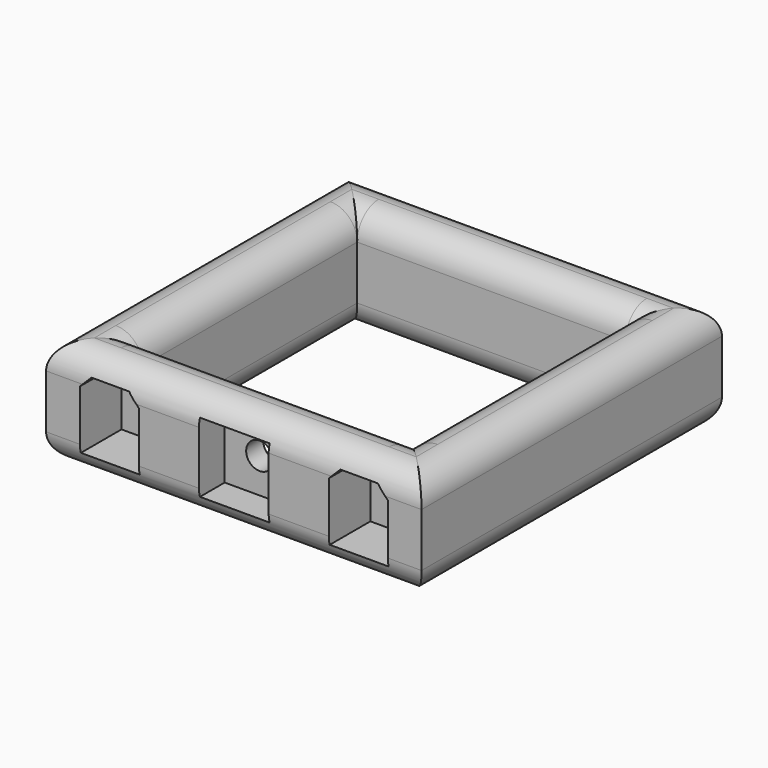
from build123d import *

# Parameters (mm, degrees)
F0_W         = 70
F0_H         = 70
F0_W_2       = 50
F0_H_2       = 50
F1_DEPTH     = 20
F2_W         = 13
F2_H         = 13
F3_DEPTH     = 6
F4_T1_DEPTH  = 95
F4_T3_DEPTH  = 95
F4_T5_DEPTH  = 50
F4_T7_DEPTH  = 50
F4_T13_DEPTH = 62.5
F4_T17_DEPTH = 62.5
F4_T24_DEPTH = 62.5
F4_T28_DEPTH = 62.5
F4_T35_DEPTH = 62.5
F4_T39_DEPTH = 62.5
F4_T46_DEPTH = 62.5
F4_T50_DEPTH = 62.5
F4_T57_DEPTH = 62.5
F4_T61_DEPTH = 62.5
F4_T68_DEPTH = 62.5
F4_T72_DEPTH = 62.5
F4_T79_DEPTH = 62.5
F4_T83_DEPTH = 62.5
F4_T90_DEPTH = 62.5
F4_T94_DEPTH = 62.5
F5_R         = 2.5
F6_DEPTH     = 25
F7_W         = 11
F7_H         = 13
F8_DEPTH     = 9.7
F9_SIZE      = 2
F10_SIZE     = 2


# Not quite as in the source:
# - a fillet or chamfer that OpenCascade refuses, or shapes differently, is made with other operations: its cross-section is extruded or revolved along the edge and cut away or added


with BuildPart() as f1:
    # F0 (on Top) → F1 (new body)
    with BuildSketch(Plane.XY):
        with Locations((7.0071799593, -0.6538340822)):
            Rectangle(F0_W, F0_H)
        with Locations((7.0071799593, -0.6538340822)):
            Rectangle(F0_W_2, F0_H_2, mode=Mode.SUBTRACT)
    extrude(amount=F1_DEPTH)

    # F2 (on face) → F3 (cut)
    with BuildSketch(Plane.XZ.offset(35.6538340822)):
        with Locations((7.0071799593, 10)):
            Rectangle(F2_W, F2_H)
    extrude(amount=-F3_DEPTH, mode=Mode.SUBTRACT)

    # F4: fillet of radius 5 on 16 edges, made by hand

    # F4_s2 → F4_t1 (cut)
    with BuildSketch(Plane.XZ.offset(-46.8461659178)):
        with BuildLine():
            ThreePointArc((42.0071799593, 5), (40.5427138653, 1.4644660941), (37.0071799593, 0))
            Line((37.0071799593, 0), (42.0071799593, 0))
            Line((42.0071799593, 0), (42.0071799593, 5))
        make_face()
        with BuildLine():
            ThreePointArc((42.0071799593, 15), (40.5427138653, 18.5355339059), (37.0071799593, 20))
            Line((37.0071799593, 20), (42.0071799593, 20))
            Line((42.0071799593, 20), (42.0071799593, 15))
        make_face()
        with BuildLine():
            ThreePointArc((-22.9928200407, 0), (-26.5283539466, 1.4644660941), (-27.9928200407, 5))
            Line((-27.9928200407, 5), (-27.9928200407, 0))
            Line((-27.9928200407, 0), (-22.9928200407, 0))
        make_face()
        with BuildLine():
            ThreePointArc((-22.9928200407, 20), (-26.5283539466, 18.5355339059), (-27.9928200407, 15))
            Line((-27.9928200407, 15), (-27.9928200407, 20))
            Line((-27.9928200407, 20), (-22.9928200407, 20))
        make_face()
    extrude(amount=F4_T1_DEPTH, mode=Mode.SUBTRACT)

    # F4_s4 → F4_t3 (cut)
    with BuildSketch(Plane.YZ.offset(-40.4928200407)):
        with BuildLine():
            ThreePointArc((-35.6538340822, 5), (-34.1893679881, 1.4644660941), (-30.6538340822, 0))
            Line((-30.6538340822, 0), (-35.6538340822, 0))
            Line((-35.6538340822, 0), (-35.6538340822, 5))
        make_face()
        with BuildLine():
            ThreePointArc((-35.6538340822, 15), (-34.1893679881, 18.5355339059), (-30.6538340822, 20))
            Line((-30.6538340822, 20), (-35.6538340822, 20))
            Line((-35.6538340822, 20), (-35.6538340822, 15))
        make_face()
        with BuildLine():
            ThreePointArc((34.3461659178, 5), (32.8816998237, 1.4644660941), (29.3461659178, 0))
            Line((29.3461659178, 0), (34.3461659178, 0))
            Line((34.3461659178, 0), (34.3461659178, 5))
        make_face()
        with BuildLine():
            ThreePointArc((34.3461659178, 15), (32.8816998237, 18.5355339059), (29.3461659178, 20))
            Line((29.3461659178, 20), (34.3461659178, 20))
            Line((34.3461659178, 20), (34.3461659178, 15))
        make_face()
    extrude(amount=F4_T3_DEPTH, mode=Mode.SUBTRACT)

    # F4_s6 → F4_t5 (cut)
    with BuildSketch(Plane.XZ.offset(-24.3461659178)):
        with BuildLine():
            ThreePointArc((-22.9928200407, 0), (-19.4572861347, 1.4644660941), (-17.9928200407, 5))
            Line((-17.9928200407, 5), (-17.9928200407, 0))
            Line((-17.9928200407, 0), (-22.9928200407, 0))
        make_face()
        with BuildLine():
            ThreePointArc((37.0071799593, 0), (33.4716460534, 1.4644660941), (32.0071799593, 5))
            Line((32.0071799593, 5), (32.0071799593, 0))
            Line((32.0071799593, 0), (37.0071799593, 0))
        make_face()
        with BuildLine():
            ThreePointArc((-22.9928200407, 20), (-19.4572861347, 18.5355339059), (-17.9928200407, 15))
            Line((-17.9928200407, 15), (-17.9928200407, 20))
            Line((-17.9928200407, 20), (-22.9928200407, 20))
        make_face()
        with BuildLine():
            ThreePointArc((37.0071799593, 20), (33.4716460534, 18.5355339059), (32.0071799593, 15))
            Line((32.0071799593, 15), (32.0071799593, 20))
            Line((32.0071799593, 20), (37.0071799593, 20))
        make_face()
    extrude(amount=F4_T5_DEPTH, mode=Mode.SUBTRACT)

    # F4_s8 → F4_t7 (cut)
    with BuildSketch(Plane.YZ.offset(-17.9928200407)):
        with BuildLine():
            ThreePointArc((29.3461659178, 0), (25.8106320119, 1.4644660941), (24.3461659178, 5))
            Line((24.3461659178, 5), (24.3461659178, 0))
            Line((24.3461659178, 0), (29.3461659178, 0))
        make_face()
        with BuildLine():
            ThreePointArc((-30.6538340822, 0), (-27.1183001763, 1.4644660941), (-25.6538340822, 5))
            Line((-25.6538340822, 5), (-25.6538340822, 0))
            Line((-25.6538340822, 0), (-30.6538340822, 0))
        make_face()
        with BuildLine():
            ThreePointArc((29.3461659178, 20), (25.8106320119, 18.5355339059), (24.3461659178, 15))
            Line((24.3461659178, 15), (24.3461659178, 20))
            Line((24.3461659178, 20), (29.3461659178, 20))
        make_face()
        with BuildLine():
            ThreePointArc((-30.6538340822, 20), (-27.1183001763, 18.5355339059), (-25.6538340822, 15))
            Line((-25.6538340822, 15), (-25.6538340822, 20))
            Line((-25.6538340822, 20), (-30.6538340822, 20))
        make_face()
    extrude(amount=F4_T7_DEPTH, mode=Mode.SUBTRACT)


with BuildPart() as f4_tool11:
    # F4_s12 → F4_t13 (new body)
    with BuildSketch(Plane.XZ.offset(38.1538340822)):
        with BuildLine():
            ThreePointArc((-22.9928200407, 0), (-19.4572861347, 1.4644660941), (-17.9928200407, 5))
            Line((-17.9928200407, 5), (-17.9928200407, 0))
            Line((-17.9928200407, 0), (-22.9928200407, 0))
        make_face()
    extrude(amount=-F4_T13_DEPTH)

    split(bisect_by=Plane.XZ.offset(25.6538340822), keep=Keep.TOP)


with BuildPart() as f4_tool15:
    # F4_s16 → F4_t17 (new body)
    with BuildSketch(Plane.YZ.offset(32.0071799593)):
        with BuildLine():
            ThreePointArc((-30.6538340822, 0), (-27.1183001763, 1.4644660941), (-25.6538340822, 5))
            Line((-25.6538340822, 5), (-25.6538340822, 0))
            Line((-25.6538340822, 0), (-30.6538340822, 0))
        make_face()
    extrude(amount=-F4_T17_DEPTH)

    split(bisect_by=Plane.YZ.offset(-17.9928200407), keep=Keep.BOTTOM)


with BuildPart() as f4_tool11_1:
    add(f4_tool11.part)

    # F4_t19: intersect F4_tool15
    add(f4_tool15.part, mode=Mode.INTERSECT)


with BuildPart() as f1_1:
    add(f1.part)

    # F4_t9: cut F4_tool11
    add(f4_tool11_1.part, mode=Mode.SUBTRACT)


with BuildPart() as f4_tool22:
    # F4_s23 → F4_t24 (new body)
    with BuildSketch(Plane.XZ.offset(25.6538340822)):
        with BuildLine():
            ThreePointArc((-22.9928200407, 0), (-19.4572861347, 1.4644660941), (-17.9928200407, 5))
            Line((-17.9928200407, 5), (-17.9928200407, 0))
            Line((-17.9928200407, 0), (-22.9928200407, 0))
        make_face()
    extrude(amount=-F4_T24_DEPTH)

    split(bisect_by=Plane.XZ.offset(-24.3461659178), keep=Keep.BOTTOM)


with BuildPart() as f4_tool26:
    # F4_s27 → F4_t28 (new body)
    with BuildSketch(Plane.YZ.offset(-30.4928200407)):
        with BuildLine():
            ThreePointArc((29.3461659178, 0), (25.8106320119, 1.4644660941), (24.3461659178, 5))
            Line((24.3461659178, 5), (24.3461659178, 0))
            Line((24.3461659178, 0), (29.3461659178, 0))
        make_face()
    extrude(amount=F4_T28_DEPTH)

    split(bisect_by=Plane.YZ.offset(-17.9928200407), keep=Keep.BOTTOM)


with BuildPart() as f4_tool22_1:
    add(f4_tool22.part)

    # F4_t30: intersect F4_tool26
    add(f4_tool26.part, mode=Mode.INTERSECT)


with BuildPart() as f1_2:
    add(f1_1.part)

    # F4_t20: cut F4_tool22
    add(f4_tool22_1.part, mode=Mode.SUBTRACT)


with BuildPart() as f4_tool33:
    # F4_s34 → F4_t35 (new body)
    with BuildSketch(Plane.YZ.offset(-17.9928200407)):
        with BuildLine():
            ThreePointArc((29.3461659178, 0), (25.8106320119, 1.4644660941), (24.3461659178, 5))
            Line((24.3461659178, 5), (24.3461659178, 0))
            Line((24.3461659178, 0), (29.3461659178, 0))
        make_face()
    extrude(amount=F4_T35_DEPTH)

    split(bisect_by=Plane.YZ.offset(32.0071799593), keep=Keep.TOP)


with BuildPart() as f4_tool37:
    # F4_s38 → F4_t39 (new body)
    with BuildSketch(Plane.XZ.offset(-36.8461659178)):
        with BuildLine():
            ThreePointArc((37.0071799593, 0), (33.4716460534, 1.4644660941), (32.0071799593, 5))
            Line((32.0071799593, 5), (32.0071799593, 0))
            Line((32.0071799593, 0), (37.0071799593, 0))
        make_face()
    extrude(amount=F4_T39_DEPTH)

    split(bisect_by=Plane.XZ.offset(-24.3461659178), keep=Keep.BOTTOM)


with BuildPart() as f4_tool33_1:
    add(f4_tool33.part)

    # F4_t41: intersect F4_tool37
    add(f4_tool37.part, mode=Mode.INTERSECT)


with BuildPart() as f1_3:
    add(f1_2.part)

    # F4_t31: cut F4_tool33
    add(f4_tool33_1.part, mode=Mode.SUBTRACT)


with BuildPart() as f4_tool44:
    # F4_s45 → F4_t46 (new body)
    with BuildSketch(Plane.XZ.offset(-24.3461659178)):
        with BuildLine():
            ThreePointArc((37.0071799593, 0), (33.4716460534, 1.4644660941), (32.0071799593, 5))
            Line((32.0071799593, 5), (32.0071799593, 0))
            Line((32.0071799593, 0), (37.0071799593, 0))
        make_face()
    extrude(amount=F4_T46_DEPTH)

    split(bisect_by=Plane.XZ.offset(25.6538340822), keep=Keep.TOP)


with BuildPart() as f4_tool48:
    # F4_s49 → F4_t50 (new body)
    with BuildSketch(Plane.YZ.offset(44.5071799593)):
        with BuildLine():
            ThreePointArc((-30.6538340822, 0), (-27.1183001763, 1.4644660941), (-25.6538340822, 5))
            Line((-25.6538340822, 5), (-25.6538340822, 0))
            Line((-25.6538340822, 0), (-30.6538340822, 0))
        make_face()
    extrude(amount=-F4_T50_DEPTH)

    split(bisect_by=Plane.YZ.offset(32.0071799593), keep=Keep.TOP)


with BuildPart() as f4_tool44_1:
    add(f4_tool44.part)

    # F4_t52: intersect F4_tool48
    add(f4_tool48.part, mode=Mode.INTERSECT)


with BuildPart() as f1_4:
    add(f1_3.part)

    # F4_t42: cut F4_tool44
    add(f4_tool44_1.part, mode=Mode.SUBTRACT)


with BuildPart() as f4_tool55:
    # F4_s56 → F4_t57 (new body)
    with BuildSketch(Plane.XZ.offset(38.1538340822)):
        with BuildLine():
            ThreePointArc((-22.9928200407, 20), (-19.4572861347, 18.5355339059), (-17.9928200407, 15))
            Line((-17.9928200407, 15), (-17.9928200407, 20))
            Line((-17.9928200407, 20), (-22.9928200407, 20))
        make_face()
    extrude(amount=-F4_T57_DEPTH)

    split(bisect_by=Plane.XZ.offset(25.6538340822), keep=Keep.TOP)


with BuildPart() as f4_tool59:
    # F4_s60 → F4_t61 (new body)
    with BuildSketch(Plane.YZ.offset(32.0071799593)):
        with BuildLine():
            ThreePointArc((-30.6538340822, 20), (-27.1183001763, 18.5355339059), (-25.6538340822, 15))
            Line((-25.6538340822, 15), (-25.6538340822, 20))
            Line((-25.6538340822, 20), (-30.6538340822, 20))
        make_face()
    extrude(amount=-F4_T61_DEPTH)

    split(bisect_by=Plane.YZ.offset(-17.9928200407), keep=Keep.BOTTOM)


with BuildPart() as f4_tool55_1:
    add(f4_tool55.part)

    # F4_t63: intersect F4_tool59
    add(f4_tool59.part, mode=Mode.INTERSECT)


with BuildPart() as f1_5:
    add(f1_4.part)

    # F4_t53: cut F4_tool55
    add(f4_tool55_1.part, mode=Mode.SUBTRACT)


with BuildPart() as f4_tool66:
    # F4_s67 → F4_t68 (new body)
    with BuildSketch(Plane.XZ.offset(25.6538340822)):
        with BuildLine():
            ThreePointArc((-22.9928200407, 20), (-19.4572861347, 18.5355339059), (-17.9928200407, 15))
            Line((-17.9928200407, 15), (-17.9928200407, 20))
            Line((-17.9928200407, 20), (-22.9928200407, 20))
        make_face()
    extrude(amount=-F4_T68_DEPTH)

    split(bisect_by=Plane.XZ.offset(-24.3461659178), keep=Keep.BOTTOM)


with BuildPart() as f4_tool70:
    # F4_s71 → F4_t72 (new body)
    with BuildSketch(Plane.YZ.offset(-30.4928200407)):
        with BuildLine():
            ThreePointArc((29.3461659178, 20), (25.8106320119, 18.5355339059), (24.3461659178, 15))
            Line((24.3461659178, 15), (24.3461659178, 20))
            Line((24.3461659178, 20), (29.3461659178, 20))
        make_face()
    extrude(amount=F4_T72_DEPTH)

    split(bisect_by=Plane.YZ.offset(-17.9928200407), keep=Keep.BOTTOM)


with BuildPart() as f4_tool66_1:
    add(f4_tool66.part)

    # F4_t74: intersect F4_tool70
    add(f4_tool70.part, mode=Mode.INTERSECT)


with BuildPart() as f1_6:
    add(f1_5.part)

    # F4_t64: cut F4_tool66
    add(f4_tool66_1.part, mode=Mode.SUBTRACT)


with BuildPart() as f4_tool77:
    # F4_s78 → F4_t79 (new body)
    with BuildSketch(Plane.YZ.offset(-17.9928200407)):
        with BuildLine():
            ThreePointArc((29.3461659178, 20), (25.8106320119, 18.5355339059), (24.3461659178, 15))
            Line((24.3461659178, 15), (24.3461659178, 20))
            Line((24.3461659178, 20), (29.3461659178, 20))
        make_face()
    extrude(amount=F4_T79_DEPTH)

    split(bisect_by=Plane.YZ.offset(32.0071799593), keep=Keep.TOP)


with BuildPart() as f4_tool81:
    # F4_s82 → F4_t83 (new body)
    with BuildSketch(Plane.XZ.offset(-36.8461659178)):
        with BuildLine():
            ThreePointArc((37.0071799593, 20), (33.4716460534, 18.5355339059), (32.0071799593, 15))
            Line((32.0071799593, 15), (32.0071799593, 20))
            Line((32.0071799593, 20), (37.0071799593, 20))
        make_face()
    extrude(amount=F4_T83_DEPTH)

    split(bisect_by=Plane.XZ.offset(-24.3461659178), keep=Keep.BOTTOM)


with BuildPart() as f4_tool77_1:
    add(f4_tool77.part)

    # F4_t85: intersect F4_tool81
    add(f4_tool81.part, mode=Mode.INTERSECT)


with BuildPart() as f1_7:
    add(f1_6.part)

    # F4_t75: cut F4_tool77
    add(f4_tool77_1.part, mode=Mode.SUBTRACT)


with BuildPart() as f4_tool88:
    # F4_s89 → F4_t90 (new body)
    with BuildSketch(Plane.XZ.offset(-24.3461659178)):
        with BuildLine():
            ThreePointArc((37.0071799593, 20), (33.4716460534, 18.5355339059), (32.0071799593, 15))
            Line((32.0071799593, 15), (32.0071799593, 20))
            Line((32.0071799593, 20), (37.0071799593, 20))
        make_face()
    extrude(amount=F4_T90_DEPTH)

    split(bisect_by=Plane.XZ.offset(25.6538340822), keep=Keep.TOP)


with BuildPart() as f4_tool92:
    # F4_s93 → F4_t94 (new body)
    with BuildSketch(Plane.YZ.offset(44.5071799593)):
        with BuildLine():
            ThreePointArc((-30.6538340822, 20), (-27.1183001763, 18.5355339059), (-25.6538340822, 15))
            Line((-25.6538340822, 15), (-25.6538340822, 20))
            Line((-25.6538340822, 20), (-30.6538340822, 20))
        make_face()
    extrude(amount=-F4_T94_DEPTH)

    split(bisect_by=Plane.YZ.offset(32.0071799593), keep=Keep.TOP)


with BuildPart() as f4_tool88_1:
    add(f4_tool88.part)

    # F4_t96: intersect F4_tool92
    add(f4_tool92.part, mode=Mode.INTERSECT)


with BuildPart() as f1_8:
    add(f1_7.part)

    # F4_t86: cut F4_tool88
    add(f4_tool88_1.part, mode=Mode.SUBTRACT)

    # F5 (on face) → F6 (cut)
    with BuildSketch(Plane.XZ.offset(29.6538340822)):
        with Locations((7.0071799593, 10)):
            Circle(F5_R)
    extrude(amount=-F6_DEPTH, mode=Mode.SUBTRACT)

    # F7 (on face) → F8 (cut)
    with BuildSketch(Plane.XZ.offset(35.6538340822)):
        with Locations((-16.1928200407, 10)):
            Rectangle(F7_W, F7_H)
        with Locations((30.2071799593, 10)):
            Rectangle(F7_W, F7_H)
    extrude(amount=-F8_DEPTH, mode=Mode.SUBTRACT)

    # F9
    f9_edges = [f1_8.edges().sort_by_distance(p)[0] for p in [
        (-21.69282, -30.688682, 16.5),
        (-10.69282, -30.688682, 16.5),
    ]]
    chamfer(f9_edges, length=F9_SIZE)

    # F10
    f10_edges = [f1_8.edges().sort_by_distance(p)[0] for p in [
        (35.70718, -30.688682, 16.5),
        (24.70718, -30.688682, 16.5),
    ]]
    chamfer(f10_edges, length=F10_SIZE)


solid = f1_8.part
